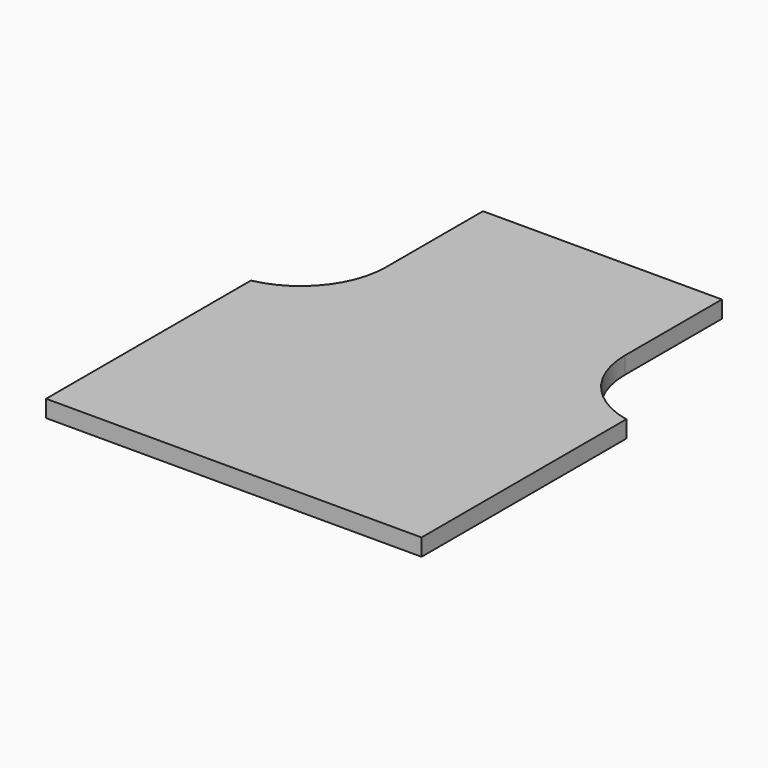
from build123d import *

# Parameters (mm, degrees)
F1_DEPTH    = 5
F2_T1_DEPTH = 5


# Not quite as in the source:
# - a fillet or chamfer that OpenCascade refuses, or shapes differently, is made with other operations: its cross-section is extruded or revolved along the edge and cut away or added


with BuildPart() as f1:
    # F0 (on Top) → F1 (new body)
    with BuildSketch(Plane.XY):
        Polygon((35, 135), (-35, 135), (-35, 75), (-55, 75), (-55, 0), (55, 0), (55, 75), (35, 75), align=None)
    extrude(amount=F1_DEPTH)

    # F2: fillet of radius 25 on 2 edges, made by hand

    # F2_s2 → F2_t1 (join)
    with BuildSketch(Plane.XY):
        with BuildLine():
            ThreePointArc((-35, 99.4948974278), (-40.635083269, 83.683509127), (-55, 75))
            Line((-55, 75), (-35, 75))
            Line((-35, 75), (-35, 99.4948974278))
        make_face()
        with BuildLine():
            ThreePointArc((55, 75), (40.635083269, 83.683509127), (35, 99.4948974278))
            Line((35, 99.4948974278), (35, 75))
            Line((35, 75), (55, 75))
        make_face()
    extrude(amount=F2_T1_DEPTH)


solid = f1.part
